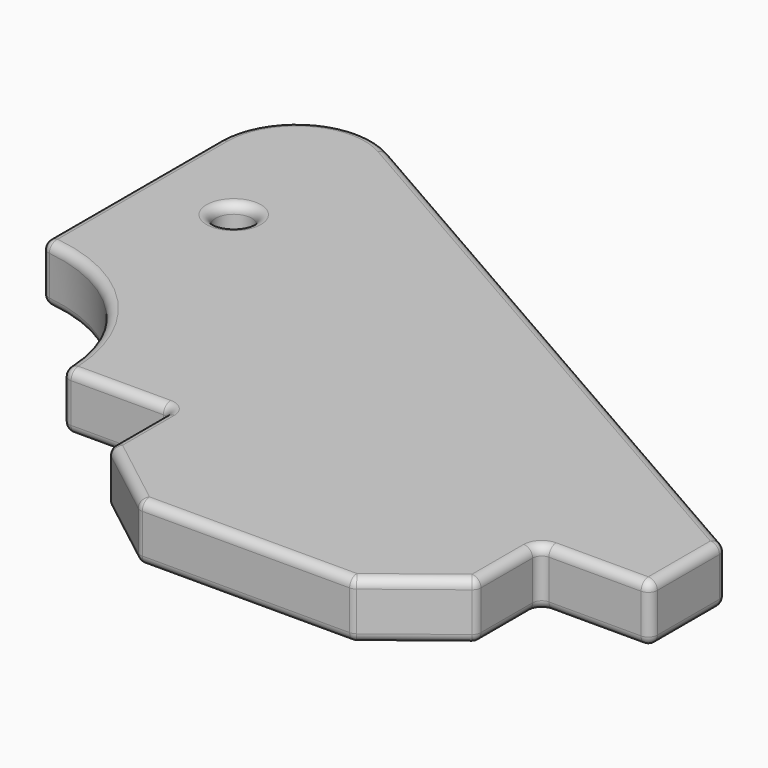
from build123d import *

# Parameters (mm, degrees)
F0_R     = 0.5
F1_DEPTH = 1.5875
F2_R     = 0.25


with BuildPart() as f1:
    # F0 (on Top) → F1 (new body)
    with BuildSketch(Plane.XY):
        with BuildLine():
            ThreePointArc((-20.32, 4.3815), (-17.4284169342, 2.9880444378), (-16.256, 0))
            Line((-16.256, 0), (-13.208, 0))
            Line((-13.208, 0), (-13.208, -2.159))
            Line((-13.208, -2.159), (-11.08075, -3.81))
            Line((-11.08075, -3.81), (-5.17525, -3.81))
            Line((-5.17525, -3.81), (-3.048, -2.159))
            Line((-3.048, -2.159), (-3.048, 0))
            Line((-3.048, 0), (0, 0))
            Line((0, 0), (0, 2.54))
            Line((0, 2.54), (-17.0995334348, 12.3433578162))
            ThreePointArc((-17.0995334348, 12.3433578162), (-19.2474502496, 12.3384695247), (-20.32, 10.4775))
            Line((-20.32, 10.4775), (-20.32, 4.3815))
        make_face()
        with Locations((-17.82, 7.8815)):
            Circle(F0_R, mode=Mode.SUBTRACT)
    extrude(amount=F1_DEPTH)

    # F2
    f2_edges = [f1.edges().sort_by_distance(p)[0] for p in [
        (-20.32, 7.4295, 1.5875),
        (-19.24745, 12.33847, 1.5875),
        (-8.549767, 7.441679, 1.5875),
        (0, 1.27, 1.5875),
        (-1.524, 0, 1.5875),
        (-3.048, -1.0795, 1.5875),
        (-4.111625, -2.9845, 1.5875),
        (-8.128, -3.81, 1.5875),
        (-12.144375, -2.9845, 1.5875),
        (-13.208, -1.0795, 1.5875),
        (-14.732, 0, 1.5875),
        (-17.428417, 2.988044, 1.5875),
        (-17.428417, 2.988044, 0),
        (-20.32, 4.3815, 0.79375),
        (0, 0, 0.79375),
        (0, 2.54, 0.79375),
        (-3.048, 0, 0.79375),
        (-3.048, -2.159, 0.79375),
        (-5.17525, -3.81, 0.79375),
        (-11.08075, -3.81, 0.79375),
        (-13.208, -2.159, 0.79375),
        (-20.32, 7.4295, 0),
        (-19.24745, 12.33847, 0),
        (-8.549767, 7.441679, 0),
        (0, 1.27, 0),
        (-13.208, -1.0795, 0),
        (-12.144375, -2.9845, 0),
        (-8.128, -3.81, 0),
        (-4.111625, -2.9845, 0),
        (-3.048, -1.0795, 0),
        (-1.524, 0, 0),
        (-16.256, 0, 0.79375),
        (-13.208, 0, 0.79375),
        (-18.32, 7.8815, 1.5875),
        (-18.32, 7.8815, 0),
        (-14.732, 0, 0),
    ]]
    fillet(f2_edges, radius=F2_R)


solid = f1.part
